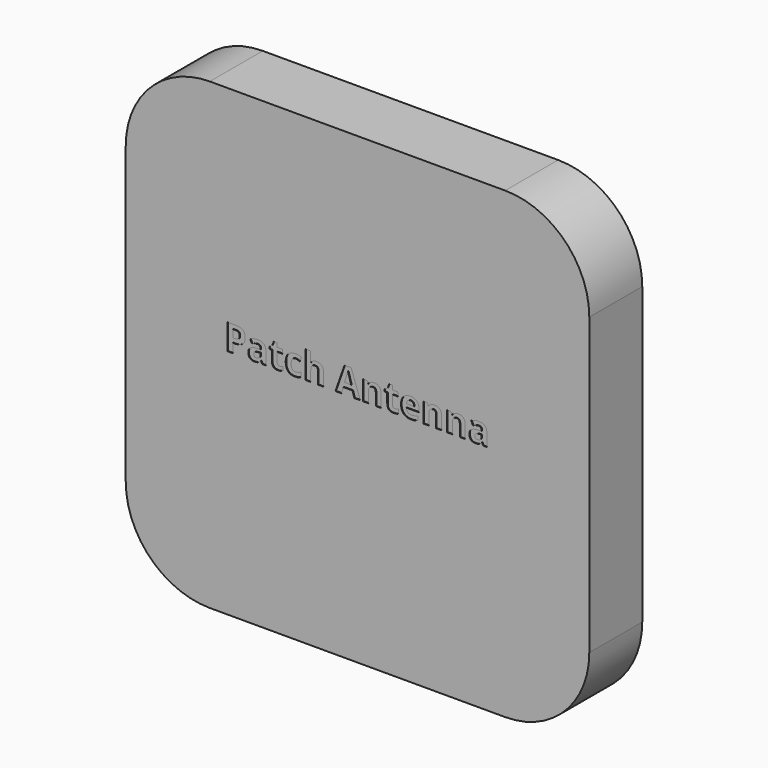
from build123d import *

# Parameters (mm, degrees)
F1_DEPTH     = 10
F2_TEXT_SIZE = 5.4220057185
F3_DEPTH     = 0.1


# Not quite as in the source:
# - Text() gives the source's letters only with a copy of the font that has no kerning and outlines rounded to 1/6400 em; it was checked with that copy


with BuildPart() as f1:
    # F0 (on Front) → F1 (new body)
    with BuildSketch(Plane.XZ):
        with BuildLine():
            ThreePointArc((35, 22.3), (31.2802561211, 31.2802561211), (22.3, 35))
            Line((22.3, 35), (-22.3, 35))
            ThreePointArc((-22.3, 35), (-31.2802561211, 31.2802561211), (-35, 22.3))
            Line((-35, 22.3), (-35, -22.3))
            ThreePointArc((-35, -22.3), (-31.2802561211, -31.2802561211), (-22.3, -35))
            Line((-22.3, -35), (22.3, -35))
            ThreePointArc((22.3, -35), (31.2802561211, -31.2802561211), (35, -22.3))
            Line((35, -22.3), (35, 22.3))
        make_face()
    extrude(amount=F1_DEPTH)

    # F2 (on face) → F3 (cut)
    with BuildSketch(Plane.XZ.offset(10)):
        with Locations((-20.1200633275, 0)):
            Text('Patch Antenna', F2_TEXT_SIZE, font='Open Sans', font_style=FontStyle.BOLD, text_align=(TextAlign.LEFT, TextAlign.BOTTOM))
    extrude(amount=-F3_DEPTH, mode=Mode.SUBTRACT)


solid = f1.part
